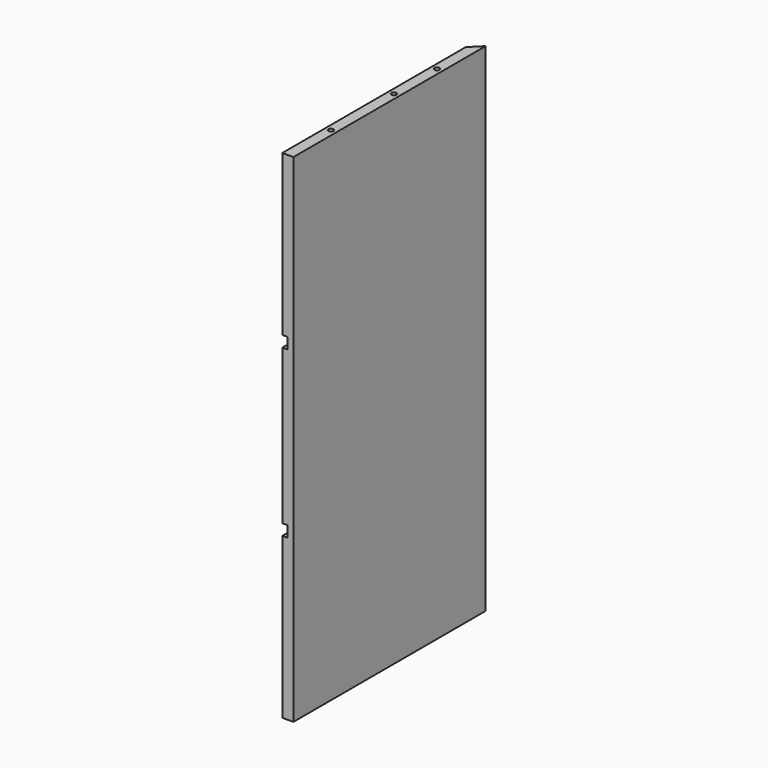
from build123d import *

# Parameters (mm, degrees)
F0_W           = 390
F0_H           = 260
F0_H_2         = 251
F0_H_3         = 18
F1_DEPTH       = 18
F2_DEPTH       = 8
F3_SIZE2       = 17.99999
F3_SIZE        = 17.99999
F6_D           = 8
F6_DEPTH       = 21
F6_TIP         = 2.4034424761
F6_ON_F5_D     = 8
F6_ON_F5_DEPTH = 21
F6_ON_F5_TIP   = 2.4034424761
F8_D           = 8
F8_DEPTH       = 11
F8_TIP         = 2.4034424761


# Not quite as in the source:
# - a fillet or chamfer is up to 0.001 mm smaller than in the source, because OpenCascade refuses the exact size


with BuildPart() as f1:
    # F0 (on Right) → F1 (new body)
    with BuildSketch(Plane.YZ):
        with Locations((0, 273.5)):
            Rectangle(F0_W, F0_H)
        Rectangle(F0_W, F0_H_2)
        with Locations((0, -273.5)):
            Rectangle(F0_W, F0_H)
        with Locations((0, 134.5)):
            Rectangle(F0_W, F0_H_3)
        with Locations((0, -134.5)):
            Rectangle(F0_W, F0_H_3)
    extrude(amount=F1_DEPTH)

    # F0 (on Right) → F2 (cut)
    with BuildSketch(Plane.YZ):
        with Locations((0, 134.5)):
            Rectangle(F0_W, F0_H_3)
        with Locations((0, -134.5)):
            Rectangle(F0_W, F0_H_3)
    extrude(amount=F2_DEPTH, mode=Mode.SUBTRACT)

    # F3 (size 18 and 18 in the source; OpenCascade refuses exactly that, so slightly less here)
    f3_edges = [f1.edges().sort_by_distance(p)[0] for p in [
        (0, 195, 0),
    ]]
    chamfer(f3_edges, length=F3_SIZE, length2=F3_SIZE2)

    # F6
    with Locations(Plane.XY.offset(403.5)):
        with Locations((9, 107.5), (9, 20), (9, -107.5)):
            Hole(F6_D / 2, depth=F6_DEPTH)
            with Locations((0, 0, -(F6_DEPTH + F6_TIP / 2))):  # 118° drill point
                Cone(0, F6_D / 2, F6_TIP, mode=Mode.SUBTRACT)

    # F6 on F5
    with Locations(Plane(origin=(0, 0, -403.5), x_dir=(1, 0, 0), z_dir=(0, 0, -1))):
        with Locations((9, -107.5), (9, -20), (9, 67.5)):
            Hole(F6_ON_F5_D / 2, depth=F6_ON_F5_DEPTH)
            with Locations((0, 0, -(F6_ON_F5_DEPTH + F6_ON_F5_TIP / 2))):  # 118° drill point
                Cone(0, F6_ON_F5_D / 2, F6_ON_F5_TIP, mode=Mode.SUBTRACT)

    # F8
    with Locations(Plane(origin=(0, 0, 0), x_dir=(0, 1, 0), z_dir=(-1, 0, 0))):
        with Locations((0, 134.5), (0, -134.5)):
            Hole(F8_D / 2, depth=F8_DEPTH)
            with Locations((0, 0, -(F8_DEPTH + F8_TIP / 2))):  # 118° drill point
                Cone(0, F8_D / 2, F8_TIP, mode=Mode.SUBTRACT)


solid = f1.part
